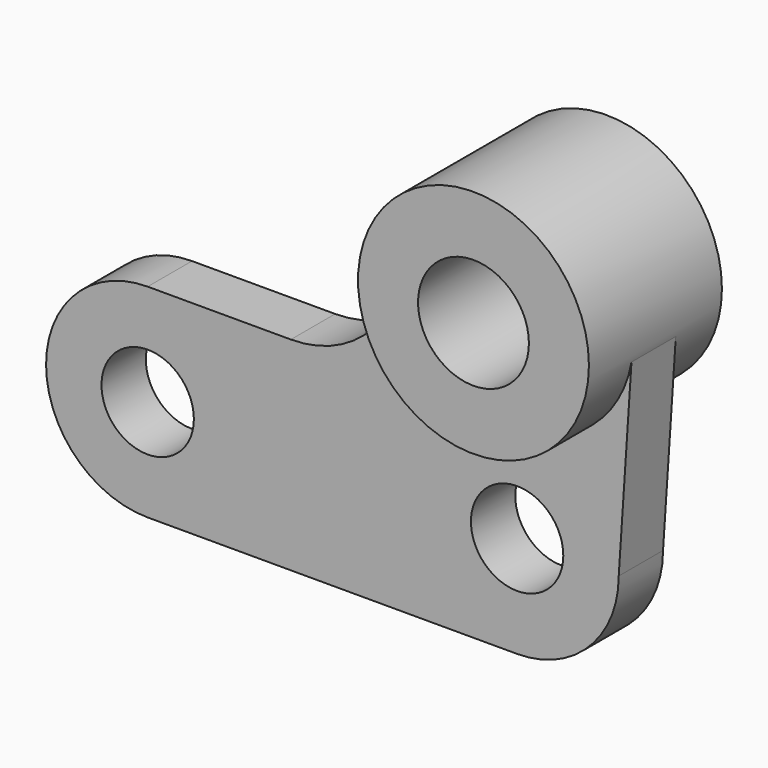
from build123d import *

# Parameters (mm, degrees)
F0_R     = 10
F1_DEPTH = 6
F2_R     = 25
F2_R_2   = 12
F3_DEPTH = 18
F4_R     = 23.9999


# Not quite as in the source:
# - a fillet or chamfer is up to 0.001 mm smaller than in the source, because OpenCascade refuses the exact size


with BuildPart() as f1:
    # F0 (on Front) → F1 (new body, symmetric)
    with BuildSketch(Plane.XZ):
        with BuildLine():
            Line((16.57635398, 22), (-38.42364602, 22))
            ThreePointArc((-38.42364602, 22), (-60.42364602, 0), (-38.42364602, -22))
            Line((-38.42364602, -22), (41.57635398, -22))
            ThreePointArc((41.57635398, -22), (57.1327031661, -15.5563491861), (63.57635398, 0))
            Line((63.57635398, 0), (66.521399326, 44.3432825568))
            ThreePointArc((66.521399326, 44.3432825568), (40.7475396611, 21.0137424406), (16.57635398, 46))
            Line((16.57635398, 46), (16.57635398, 22))
        make_face()
        with Locations((-38.42364602, 0)):
            Circle(F0_R, mode=Mode.SUBTRACT)
        with Locations((41.57635398, 0)):
            Circle(F0_R, mode=Mode.SUBTRACT)
    extrude(amount=F1_DEPTH, both=True)

    # F2 (on Front) → F3 (join, symmetric)
    with BuildSketch(Plane.XZ):
        with Locations((41.726754687, 46.0397801568)):
            Circle(F2_R)
        with Locations((41.726754687, 46.0397801568)):
            Circle(F2_R_2, mode=Mode.SUBTRACT)
    extrude(amount=F3_DEPTH, both=True)

    # F4 (radius 24 in the source; OpenCascade refuses exactly that, so slightly less here)
    f4_edges = [f1.edges().sort_by_distance(p)[0] for p in [
        (16.576354, 0, 22),
    ]]
    fillet(f4_edges, radius=F4_R)


solid = f1.part
